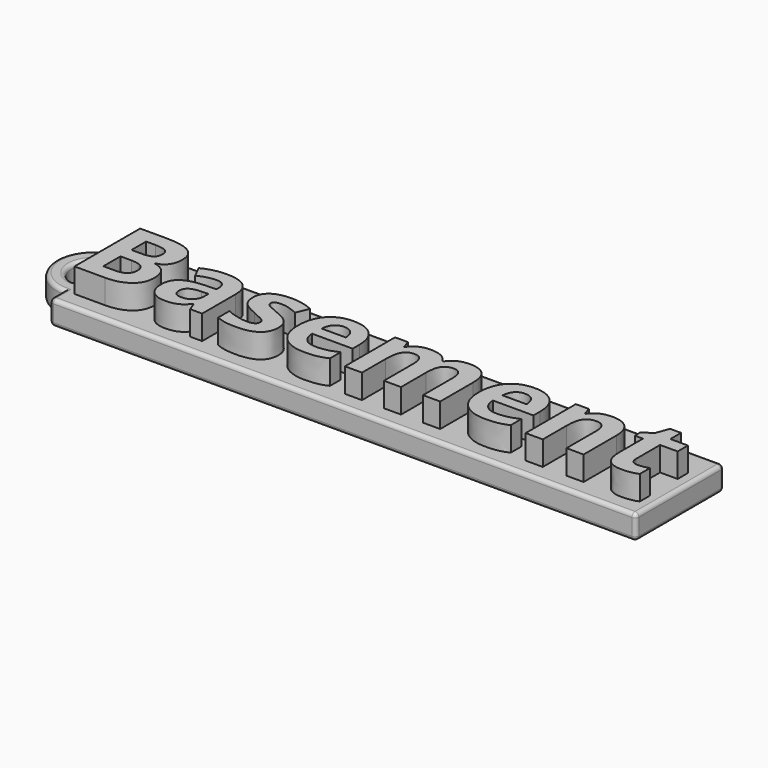
from build123d import *

# Parameters (mm, degrees)
F0_TEXT_SIZE = 15.05835855
F1_DEPTH     = 3.175
F3_DEPTH     = 3.175
F4_R         = 0.508


# Not quite as in the source:
# - Text() gives the source's letters only with a copy of the font that has no kerning and outlines rounded to 1/6400 em; it was checked with that copy


with BuildPart() as f1:
    # F0 (on Top) → F1 (new body)
    with BuildSketch(Plane.XY):
        with Locations((-38.1, -4.9694525078)):
            Text('Basement', F0_TEXT_SIZE, font='Open Sans', font_style=FontStyle.BOLD, text_align=(TextAlign.LEFT, TextAlign.BOTTOM))
    extrude(amount=F1_DEPTH)

    # F2 (on Top) → F3 (join)
    with BuildSketch(Plane.XY):
        with BuildLine():
            Line((38.1438648328, 7.154814899), (-37.6727236435, 7.154814899))
            Line((-37.6727236435, 7.154814899), (-38.1560400128, 7.154814899))
            Line((-38.1560400128, 7.154814899), (-38.1560400128, 6.6714985296))
            Line((-38.1560400128, 6.6714985296), (-38.1560400128, 4.8202062453))
            ThreePointArc((-38.1560400128, 4.8202062453), (-43.0327349304, -0.0564886723), (-38.1560400128, -4.9331835898))
            Line((-38.1560400128, -4.9331835898), (-38.1560400128, -6.7844758742))
            Line((-38.1560400128, -6.7844758742), (-38.1560400128, -7.2677922435))
            Line((-38.1560400128, -7.2677922435), (-37.6727236435, -7.2677922435))
            Line((-37.6727236435, -7.2677922435), (38.1438648328, -7.2677922435))
            Line((38.1438648328, -7.2677922435), (38.6271812022, -7.2677922435))
            Line((38.6271812022, -7.2677922435), (38.6271812022, -6.7844758742))
            Line((38.6271812022, -6.7844758742), (38.6271812022, 6.6714985296))
            Line((38.6271812022, 6.6714985296), (38.6271812022, 7.154814899))
            Line((38.6271812022, 7.154814899), (38.1438648328, 7.154814899))
        make_face()
        with BuildLine():
            ThreePointArc((-38.1560400128, -2.9253107815), (-41.0248621221, -0.0564886723), (-38.1560400128, 2.812333437))
            Line((-38.1560400128, 2.812333437), (-38.1560400128, -2.9253107815))
        make_face(mode=Mode.SUBTRACT)
    extrude(amount=-F3_DEPTH)

    # F4
    f4_edges = [f1.edges().sort_by_distance(p)[0] for p in [
        (0.235571, 7.154815, 0),
        (0.235571, 7.154815, -3.175),
        (-38.15604, 7.154815, -1.5875),
        (-38.15604, 4.820206, -1.5875),
        (-38.15604, 5.987511, 0),
        (-43.032735, -0.056489, 0),
        (-38.15604, -6.100488, 0),
        (0.235571, -7.267792, 0),
        (38.627181, -0.056489, 0),
        (38.627181, 7.154815, -1.5875),
        (38.627181, -7.267792, -1.5875),
        (0.235571, -7.267792, -3.175),
        (38.627181, -0.056489, -3.175),
        (-38.15604, 5.987511, -3.175),
        (-43.032735, -0.056489, -3.175),
        (-38.15604, -6.100488, -3.175),
        (-38.15604, -7.267792, -1.5875),
        (-38.15604, -0.056489, -3.175),
        (-41.024862, -0.056489, -3.175),
        (-38.15604, -0.056489, 0),
        (-41.024862, -0.056489, 0),
        (-38.15604, 2.812333, -1.5875),
        (-38.15604, -2.925311, -1.5875),
    ]]
    fillet(f4_edges, radius=F4_R)


solid = f1.part
